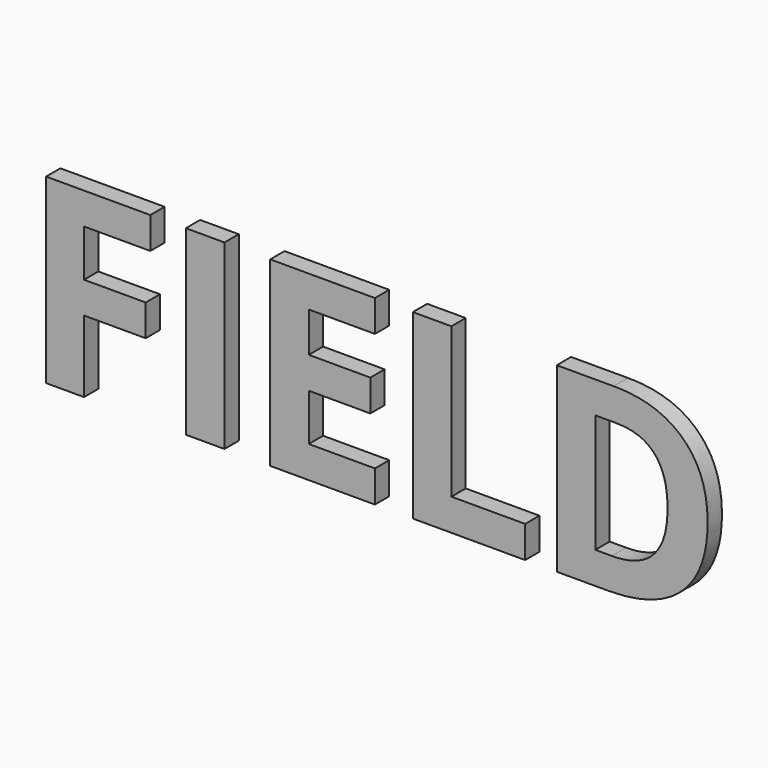
from build123d import *

# Parameters (mm, degrees)
F0_TEXT_SIZE = 542.625433041
F1_DEPTH     = 38.1


# Not quite as in the source:
# - Text() gives the source's letters only with a copy of the font that has no kerning and outlines rounded to 1/6400 em; it was checked with that copy


with BuildPart() as f1:
    # F0 (on Front) → F1 (new body)
    with BuildSketch(Plane.XZ):
        with Locations((-742.5529360771, -192.4338489771)):
            Text('FIELD', F0_TEXT_SIZE, font='Open Sans', font_style=FontStyle.BOLD, text_align=(TextAlign.LEFT, TextAlign.BOTTOM))
    extrude(amount=F1_DEPTH)


solid = f1.part
